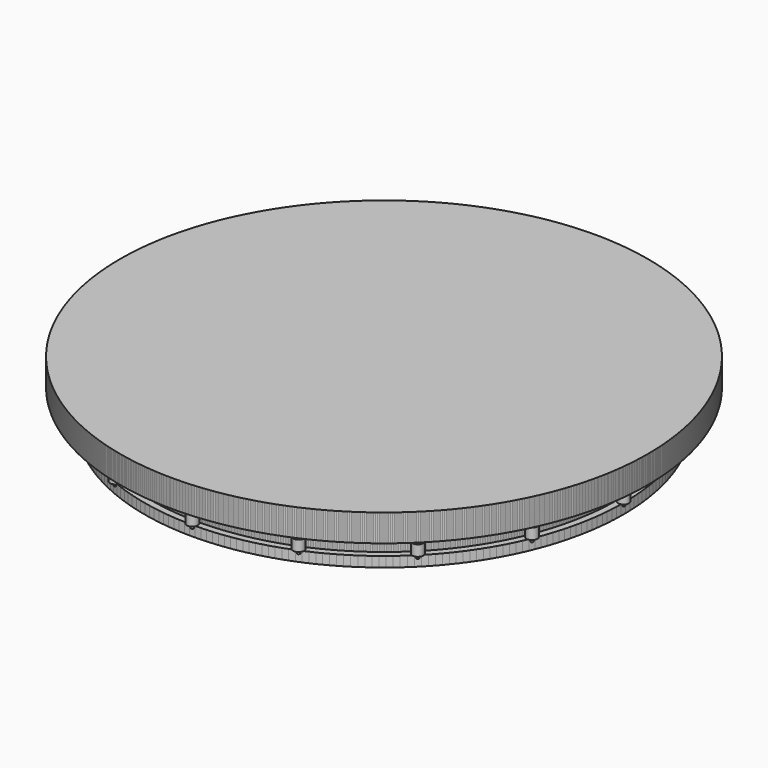
from build123d import *

# Parameters (mm, degrees)
F1_W     = 1
F1_H     = 8
F1_W_2   = 3
F5_COUNT = 16
F6_R     = 7
F7_DEPTH = 20


with BuildPart() as f2:
    # F1 (on Front) → F2 (revolve)
    with BuildSketch(Plane.XZ):
        Polygon((194.0861491203, -20), (194.0861491203, 0), (0, 0), (0, -45), (176.1861491203, -45), (176.1861491203, -39.5), (176.1861491203, -37.5), (171.1861491203, -37.5), (171.1861491203, -27.5), (176.1861491203, -27.5), (176.1861491203, -25.5), (176.1861491203, -20), align=None)
    revolve(axis=Axis((0, 0, 0), (0, 0, 1)))


with BuildPart() as f3:
    # F1 (on Front) → F3 (revolve)
    with BuildSketch(Plane.XZ):
        Polygon((177.1861491203, -25.5), (176.1861491203, -25.5), (176.1861491203, -27.5), (176.1861491203, -28.5), (177.1861491203, -28.5), align=None)
        with Locations((176.6861491203, -32.5)):
            Rectangle(F1_W, F1_H)
        Polygon((176.1861491203, -37.5), (176.1861491203, -39.5), (177.1861491203, -39.5), (177.1861491203, -36.5), (176.1861491203, -36.5), align=None)
    revolve(axis=Axis((176.1861491203, 0, -32.5), (0, 0, 1)))


with BuildPart() as f4:
    # F1 (on Front) → F4 (revolve)
    with BuildSketch(Plane.XZ):
        with Locations((178.6861491203, -32.5)):
            Rectangle(F1_W_2, F1_H)
    revolve(axis=Axis((176.1861491203, 0, -32.5), (0, 0, 1)))


with BuildPart() as f5_1:
    # F5: instance of F4
    add(f4.part.rotate(Axis((0, 0, -22.5), (0, 0, 1)), 1 * 360 / F5_COUNT))


with BuildPart() as f5_2:
    # F5: instance of F4
    add(f4.part.rotate(Axis((0, 0, -22.5), (0, 0, 1)), 2 * 360 / F5_COUNT))


with BuildPart() as f5_3:
    # F5: instance of F4
    add(f4.part.rotate(Axis((0, 0, -22.5), (0, 0, 1)), 3 * 360 / F5_COUNT))


with BuildPart() as f5_4:
    # F5: instance of F4
    add(f4.part.rotate(Axis((0, 0, -22.5), (0, 0, 1)), 4 * 360 / F5_COUNT))


with BuildPart() as f5_5:
    # F5: instance of F4
    add(f4.part.rotate(Axis((0, 0, -22.5), (0, 0, 1)), 5 * 360 / F5_COUNT))


with BuildPart() as f5_6:
    # F5: instance of F4
    add(f4.part.rotate(Axis((0, 0, -22.5), (0, 0, 1)), 6 * 360 / F5_COUNT))


with BuildPart() as f5_7:
    # F5: instance of F4
    add(f4.part.rotate(Axis((0, 0, -22.5), (0, 0, 1)), 7 * 360 / F5_COUNT))


with BuildPart() as f5_8:
    # F5: instance of F4
    add(f4.part.rotate(Axis((0, 0, -22.5), (0, 0, 1)), 8 * 360 / F5_COUNT))


with BuildPart() as f5_9:
    # F5: instance of F4
    add(f4.part.rotate(Axis((0, 0, -22.5), (0, 0, 1)), 9 * 360 / F5_COUNT))


with BuildPart() as f5_10:
    # F5: instance of F4
    add(f4.part.rotate(Axis((0, 0, -22.5), (0, 0, 1)), 10 * 360 / F5_COUNT))


with BuildPart() as f5_11:
    # F5: instance of F4
    add(f4.part.rotate(Axis((0, 0, -22.5), (0, 0, 1)), 11 * 360 / F5_COUNT))


with BuildPart() as f5_12:
    # F5: instance of F4
    add(f4.part.rotate(Axis((0, 0, -22.5), (0, 0, 1)), 12 * 360 / F5_COUNT))


with BuildPart() as f5_13:
    # F5: instance of F4
    add(f4.part.rotate(Axis((0, 0, -22.5), (0, 0, 1)), 13 * 360 / F5_COUNT))


with BuildPart() as f5_14:
    # F5: instance of F4
    add(f4.part.rotate(Axis((0, 0, -22.5), (0, 0, 1)), 14 * 360 / F5_COUNT))


with BuildPart() as f5_15:
    # F5: instance of F4
    add(f4.part.rotate(Axis((0, 0, -22.5), (0, 0, 1)), 15 * 360 / F5_COUNT))


with BuildPart() as f5_16:
    # F5: instance of F3
    add(f3.part.rotate(Axis((0, 0, -22.5), (0, 0, 1)), 1 * 360 / F5_COUNT))


with BuildPart() as f5_17:
    # F5: instance of F3
    add(f3.part.rotate(Axis((0, 0, -22.5), (0, 0, 1)), 2 * 360 / F5_COUNT))


with BuildPart() as f5_18:
    # F5: instance of F3
    add(f3.part.rotate(Axis((0, 0, -22.5), (0, 0, 1)), 3 * 360 / F5_COUNT))


with BuildPart() as f5_19:
    # F5: instance of F3
    add(f3.part.rotate(Axis((0, 0, -22.5), (0, 0, 1)), 4 * 360 / F5_COUNT))


with BuildPart() as f5_20:
    # F5: instance of F3
    add(f3.part.rotate(Axis((0, 0, -22.5), (0, 0, 1)), 5 * 360 / F5_COUNT))


with BuildPart() as f5_21:
    # F5: instance of F3
    add(f3.part.rotate(Axis((0, 0, -22.5), (0, 0, 1)), 6 * 360 / F5_COUNT))


with BuildPart() as f5_22:
    # F5: instance of F3
    add(f3.part.rotate(Axis((0, 0, -22.5), (0, 0, 1)), 7 * 360 / F5_COUNT))


with BuildPart() as f5_23:
    # F5: instance of F3
    add(f3.part.rotate(Axis((0, 0, -22.5), (0, 0, 1)), 8 * 360 / F5_COUNT))


with BuildPart() as f5_24:
    # F5: instance of F3
    add(f3.part.rotate(Axis((0, 0, -22.5), (0, 0, 1)), 9 * 360 / F5_COUNT))


with BuildPart() as f5_25:
    # F5: instance of F3
    add(f3.part.rotate(Axis((0, 0, -22.5), (0, 0, 1)), 10 * 360 / F5_COUNT))


with BuildPart() as f5_26:
    # F5: instance of F3
    add(f3.part.rotate(Axis((0, 0, -22.5), (0, 0, 1)), 11 * 360 / F5_COUNT))


with BuildPart() as f5_27:
    # F5: instance of F3
    add(f3.part.rotate(Axis((0, 0, -22.5), (0, 0, 1)), 12 * 360 / F5_COUNT))


with BuildPart() as f5_28:
    # F5: instance of F3
    add(f3.part.rotate(Axis((0, 0, -22.5), (0, 0, 1)), 13 * 360 / F5_COUNT))


with BuildPart() as f5_29:
    # F5: instance of F3
    add(f3.part.rotate(Axis((0, 0, -22.5), (0, 0, 1)), 14 * 360 / F5_COUNT))


with BuildPart() as f5_30:
    # F5: instance of F3
    add(f3.part.rotate(Axis((0, 0, -22.5), (0, 0, 1)), 15 * 360 / F5_COUNT))


with BuildPart() as f5_31:
    # F5: instance of F2
    add(f2.part.rotate(Axis((0, 0, -22.5), (0, 0, 1)), 1 * 360 / F5_COUNT))


with BuildPart() as f5_32:
    # F5: instance of F2
    add(f2.part.rotate(Axis((0, 0, -22.5), (0, 0, 1)), 2 * 360 / F5_COUNT))


with BuildPart() as f5_33:
    # F5: instance of F2
    add(f2.part.rotate(Axis((0, 0, -22.5), (0, 0, 1)), 3 * 360 / F5_COUNT))


with BuildPart() as f5_34:
    # F5: instance of F2
    add(f2.part.rotate(Axis((0, 0, -22.5), (0, 0, 1)), 4 * 360 / F5_COUNT))


with BuildPart() as f5_35:
    # F5: instance of F2
    add(f2.part.rotate(Axis((0, 0, -22.5), (0, 0, 1)), 5 * 360 / F5_COUNT))


with BuildPart() as f5_36:
    # F5: instance of F2
    add(f2.part.rotate(Axis((0, 0, -22.5), (0, 0, 1)), 6 * 360 / F5_COUNT))


with BuildPart() as f5_37:
    # F5: instance of F2
    add(f2.part.rotate(Axis((0, 0, -22.5), (0, 0, 1)), 7 * 360 / F5_COUNT))


with BuildPart() as f5_38:
    # F5: instance of F2
    add(f2.part.rotate(Axis((0, 0, -22.5), (0, 0, 1)), 8 * 360 / F5_COUNT))


with BuildPart() as f5_39:
    # F5: instance of F2
    add(f2.part.rotate(Axis((0, 0, -22.5), (0, 0, 1)), 9 * 360 / F5_COUNT))


with BuildPart() as f5_40:
    # F5: instance of F2
    add(f2.part.rotate(Axis((0, 0, -22.5), (0, 0, 1)), 10 * 360 / F5_COUNT))


with BuildPart() as f5_41:
    # F5: instance of F2
    add(f2.part.rotate(Axis((0, 0, -22.5), (0, 0, 1)), 11 * 360 / F5_COUNT))


with BuildPart() as f5_42:
    # F5: instance of F2
    add(f2.part.rotate(Axis((0, 0, -22.5), (0, 0, 1)), 12 * 360 / F5_COUNT))


with BuildPart() as f5_43:
    # F5: instance of F2
    add(f2.part.rotate(Axis((0, 0, -22.5), (0, 0, 1)), 13 * 360 / F5_COUNT))


with BuildPart() as f5_44:
    # F5: instance of F2
    add(f2.part.rotate(Axis((0, 0, -22.5), (0, 0, 1)), 14 * 360 / F5_COUNT))


with BuildPart() as f5_45:
    # F5: instance of F2
    add(f2.part.rotate(Axis((0, 0, -22.5), (0, 0, 1)), 15 * 360 / F5_COUNT))


with BuildPart() as f7_tool:
    # F6 (on face) → F7 (new body)
    with BuildSketch(Plane(origin=(0, 0, -45), x_dir=(1, 0, 0), z_dir=(0, 0, -1))):
        Circle(F6_R)
    extrude(amount=-F7_DEPTH)


with BuildPart() as f2_1:
    add(f2.part)

    # F7: cut by f7_tool
    add(f7_tool.part, mode=Mode.SUBTRACT)


with BuildPart() as f5_31_1:
    add(f5_31.part)

    # F7: cut by f7_tool
    add(f7_tool.part, mode=Mode.SUBTRACT)


with BuildPart() as f5_32_1:
    add(f5_32.part)

    # F7: cut by f7_tool
    add(f7_tool.part, mode=Mode.SUBTRACT)


with BuildPart() as f5_33_1:
    add(f5_33.part)

    # F7: cut by f7_tool
    add(f7_tool.part, mode=Mode.SUBTRACT)


with BuildPart() as f5_34_1:
    add(f5_34.part)

    # F7: cut by f7_tool
    add(f7_tool.part, mode=Mode.SUBTRACT)


with BuildPart() as f5_35_1:
    add(f5_35.part)

    # F7: cut by f7_tool
    add(f7_tool.part, mode=Mode.SUBTRACT)


with BuildPart() as f5_36_1:
    add(f5_36.part)

    # F7: cut by f7_tool
    add(f7_tool.part, mode=Mode.SUBTRACT)


with BuildPart() as f5_37_1:
    add(f5_37.part)

    # F7: cut by f7_tool
    add(f7_tool.part, mode=Mode.SUBTRACT)


with BuildPart() as f5_38_1:
    add(f5_38.part)

    # F7: cut by f7_tool
    add(f7_tool.part, mode=Mode.SUBTRACT)


with BuildPart() as f5_39_1:
    add(f5_39.part)

    # F7: cut by f7_tool
    add(f7_tool.part, mode=Mode.SUBTRACT)


with BuildPart() as f5_40_1:
    add(f5_40.part)

    # F7: cut by f7_tool
    add(f7_tool.part, mode=Mode.SUBTRACT)


with BuildPart() as f5_41_1:
    add(f5_41.part)

    # F7: cut by f7_tool
    add(f7_tool.part, mode=Mode.SUBTRACT)


with BuildPart() as f5_42_1:
    add(f5_42.part)

    # F7: cut by f7_tool
    add(f7_tool.part, mode=Mode.SUBTRACT)


with BuildPart() as f5_43_1:
    add(f5_43.part)

    # F7: cut by f7_tool
    add(f7_tool.part, mode=Mode.SUBTRACT)


with BuildPart() as f5_44_1:
    add(f5_44.part)

    # F7: cut by f7_tool
    add(f7_tool.part, mode=Mode.SUBTRACT)


with BuildPart() as f5_45_1:
    add(f5_45.part)

    # F7: cut by f7_tool
    add(f7_tool.part, mode=Mode.SUBTRACT)


solid = Compound([f3.part, f4.part, f5_1.part, f5_2.part, f5_3.part, f5_4.part, f5_5.part, f5_6.part, f5_7.part, f5_8.part, f5_9.part, f5_10.part, f5_11.part, f5_12.part, f5_13.part, f5_14.part, f5_15.part, f5_16.part, f5_17.part, f5_18.part, f5_19.part, f5_20.part, f5_21.part, f5_22.part, f5_23.part, f5_24.part, f5_25.part, f5_26.part, f5_27.part, f5_28.part, f5_29.part, f5_30.part, f2_1.part, f5_31_1.part, f5_32_1.part, f5_33_1.part, f5_34_1.part, f5_35_1.part, f5_36_1.part, f5_37_1.part, f5_38_1.part, f5_39_1.part, f5_40_1.part, f5_41_1.part, f5_42_1.part, f5_43_1.part, f5_44_1.part, f5_45_1.part])
